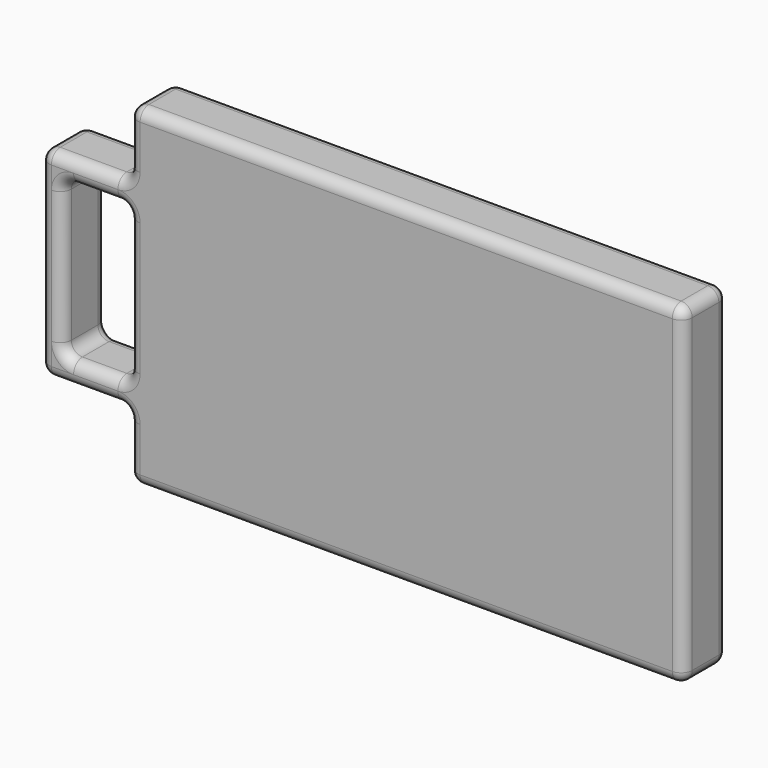
from build123d import *

# Parameters (mm, degrees)
F1_DEPTH = 25
F2_R     = 5
F3_R     = 5
F4_R     = 4.99999


# Not quite as in the source:
# - a fillet or chamfer is up to 0.001 mm smaller than in the source, because OpenCascade refuses the exact size


with BuildPart() as f1:
    # F0 (on Front) → F1 (new body)
    with BuildSketch(Plane.XZ):
        Polygon((-125, 35), (-125, 45), (-165, 45), (-165, -45), (-125, -45), (-125, -35), (-155, -35), (-155, 35), align=None)
        Polygon((125, -75), (125, 75), (-125, 75), (-125, 45), (-125, 35), (-125, -35), (-125, -45), (-125, -75), align=None)
    extrude(amount=F1_DEPTH)

    # F2
    f2_edges = [f1.edges().sort_by_distance(p)[0] for p in [
        (-125, -12.5, 45),
        (-165, -12.5, 45),
        (-165, -12.5, -45),
        (-125, -12.5, -45),
        (-125, -12.5, -35),
        (-155, -12.5, -35),
        (-155, -12.5, 35),
        (-125, -12.5, 35),
        (-125, -12.5, 75),
        (-125, -12.5, -75),
        (125, -12.5, -75),
        (125, -12.5, 75),
    ]]
    fillet(f2_edges, radius=F2_R)

    # F3
    f3_edges = [f1.edges().sort_by_distance(p)[0] for p in [
        (-145, -25, 45),
    ]]
    fillet(f3_edges, radius=F3_R)

    # F4 (radius 5 in the source; OpenCascade refuses exactly that, so slightly less here)
    f4_edges = [f1.edges().sort_by_distance(p)[0] for p in [
        (-140, -25, 35),
        (-145, 0, -45),
        (-140, 0, -35),
    ]]
    fillet(f4_edges, radius=F4_R)


solid = f1.part
